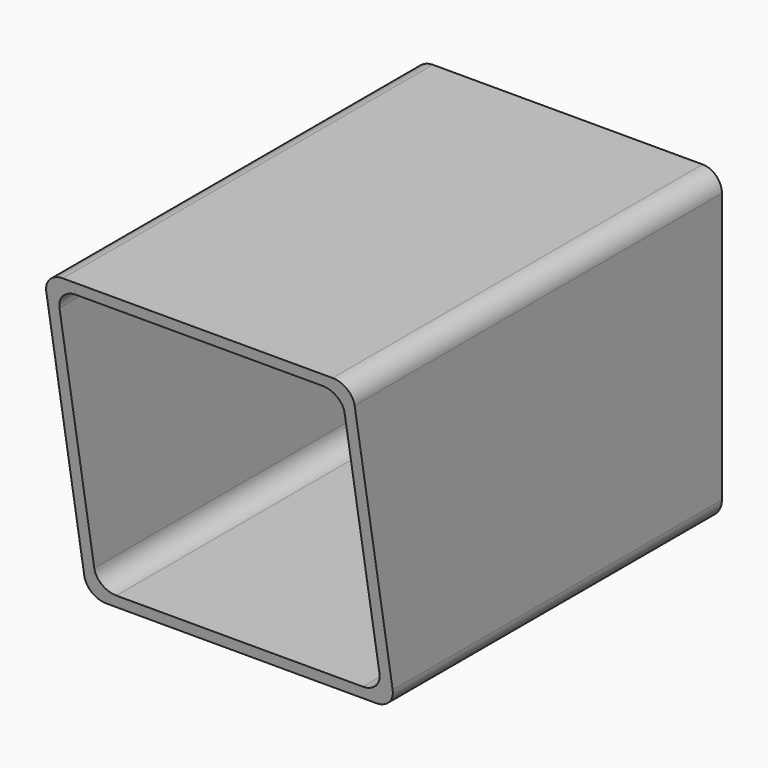
from build123d import *

# Parameters (mm, degrees)
F0_W     = 80
F0_H     = 80
F0_W_2   = 74
F0_H_2   = 74
F1_DEPTH = 120
F3_DEPTH = 80.001
F4_R     = 3
F5_DEPTH = 25
F6_R     = 5


# Not quite as in the source:
# - a feature names something its author has since deleted; it is built from what else it names


with BuildPart() as f1:
    # F0 (on Front) → F1 (new body)
    with BuildSketch(Plane.XZ):
        Rectangle(F0_W, F0_H)
        Rectangle(F0_W_2, F0_H_2, mode=Mode.SUBTRACT)
    extrude(amount=F1_DEPTH)

    # F2 (on face) → F3 (cut, through all)
    with BuildSketch(Plane(origin=(-40, 0, 0), x_dir=(0, -1, 0), z_dir=(-1, 0, 0))):
        Polygon((120, -40), (120, 40), (105.8938415433, -40), align=None)
    extrude(amount=-F3_DEPTH, mode=Mode.SUBTRACT)

    # F4 (on face) → F5 (cut)
    with BuildSketch(Plane(origin=(0, 0, -40), x_dir=(1, 0, 0), z_dir=(0, 0, -1))):
        with Locations((0, 40)):
            Circle(F4_R)
    extrude(amount=-F5_DEPTH, mode=Mode.SUBTRACT)

    # F6
    f6_edges = [f1.edges().sort_by_distance(p)[0] for p in [
        (40, -60, 40),
        (40, -52.946921, -40),
        (-40, -60, 40),
        (-40, -52.946921, -40),
        (37, -59.73551, 37),
        (37, -53.211411, -37),
        (-37, -53.211411, -37),
        (-37, -59.73551, 37),
    ]]
    fillet(f6_edges, radius=F6_R)


solid = f1.part
